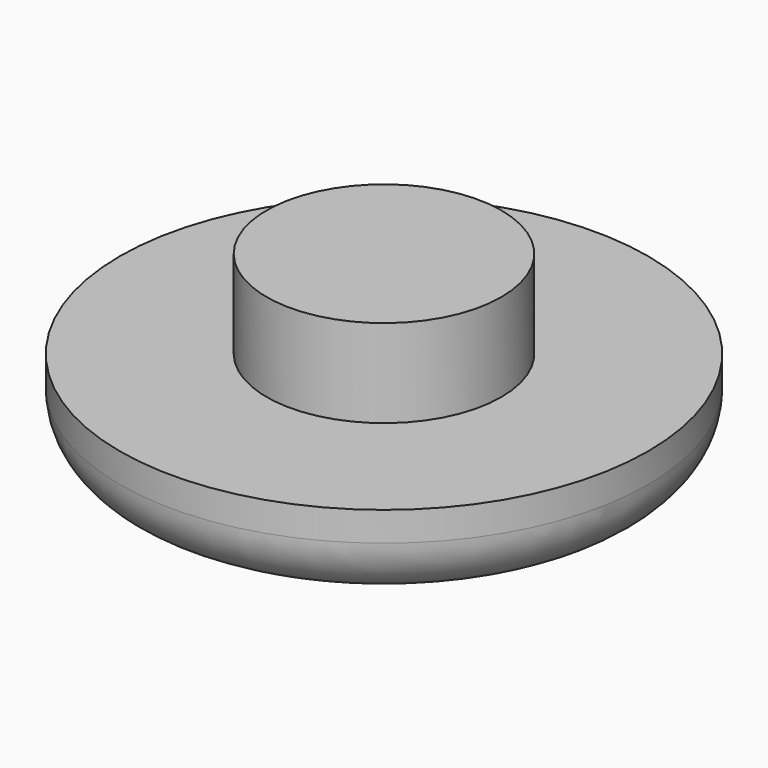
from build123d import *

# Parameters (mm, degrees)
F0_R         = 9
F1_DEPTH     = 3
F2_R         = 4
F3_DEPTH     = 3
F4_R         = 2
F5_TEXT_SIZE = 10.0039659934
F6_DEPTH     = 1.5


# Not quite as in the source:
# - Text() gives the source's letters only with a copy of the font that has no kerning and outlines rounded to 1/6400 em; it was checked with that copy


with BuildPart() as f1:
    # F0 (on Top) → F1 (new body)
    with BuildSketch(Plane.XY):
        Circle(F0_R)
    extrude(amount=F1_DEPTH)

    # F2 (on face) → F3 (join)
    with BuildSketch(Plane.XY.offset(3)):
        Circle(F2_R)
    extrude(amount=F3_DEPTH)

    # F4
    f4_edges = [f1.edges().sort_by_distance(p)[0] for p in [
        (-9, 0, 0),
    ]]
    fillet(f4_edges, radius=F4_R)

    # F5 (on face) → F6 (cut)
    with BuildSketch(Plane(origin=(0, 0, 0), x_dir=(1, 0, 0), z_dir=(0, 0, -1))):
        with Locations((-6.088126363, -3.4546660313)):
            Text('VB', F5_TEXT_SIZE, font='Open Sans', font_style=FontStyle.ITALIC, text_align=(TextAlign.LEFT, TextAlign.BOTTOM))
    extrude(amount=-F6_DEPTH, mode=Mode.SUBTRACT)


solid = f1.part
